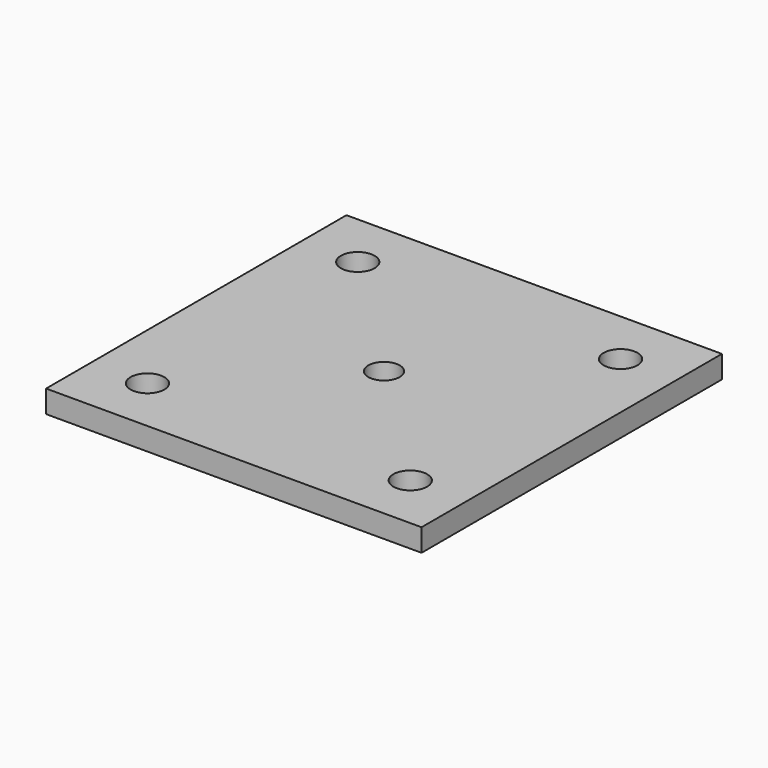
from build123d import *

# Parameters (mm, degrees)
F0_W     = 50
F0_H     = 50
F0_R     = 2
F0_R_2   = 2.1
F1_DEPTH = 3
F2_D     = 4.5


# Not quite as in the source:
# - a feature names something its author has since deleted; it is built from what else it names


with BuildPart() as f1:
    # F0 (on Top) → F1 (new body)
    with BuildSketch(Plane.XY):
        with Locations((-3.725e-07, 2.55218e-05)):
            Rectangle(F0_W, F0_H)
        with Locations((-17.5000003725, -17.4999744782)):
            Circle(F0_R, mode=Mode.SUBTRACT)
        with Locations((17.4999996275, -17.4999744782)):
            Circle(F0_R, mode=Mode.SUBTRACT)
        Circle(F0_R_2, mode=Mode.SUBTRACT)
        with Locations((-17.5000003725, 17.5000255218)):
            Circle(F0_R, mode=Mode.SUBTRACT)
        with Locations((17.4999996275, 17.5000255218)):
            Circle(F0_R, mode=Mode.SUBTRACT)
    extrude(amount=F1_DEPTH)

    # F2 (through all)
    with Locations(Plane(origin=(0, 0, 0), x_dir=(1, 0, 0), z_dir=(0, 0, -1))):
        with Locations((-17.5000003725, 17.4999744782), (-17.5000003725, -17.5000255218), (17.4999996275, -17.5000255218), (17.4999996275, 17.4999744782)):
            Hole(F2_D / 2)


solid = f1.part
